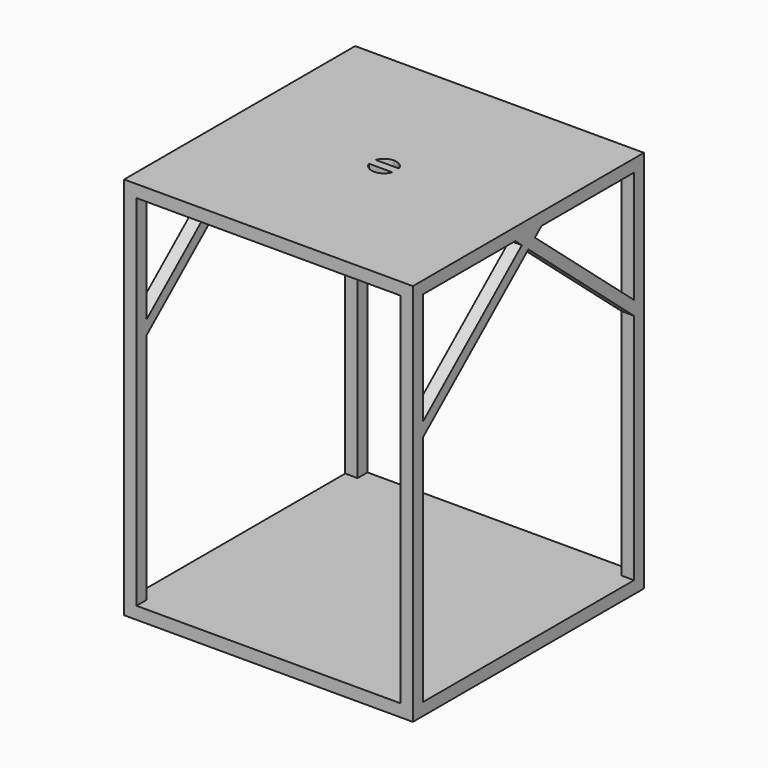
from build123d import *

# Parameters (mm, degrees)
F0_W     = 35
F0_H     = 70
F1_DEPTH = 3
F3_DEPTH = 3
F5_DEPTH = 3


# Not quite as in the source:
# - a feature names something its author has since deleted; it is built from what else it names


with BuildPart() as f1:
    # F0 (on Top) → F1 (new body)
    with BuildSketch(Plane.XY):
        with Locations((-17.5, 35)):
            Rectangle(F0_W, F0_H)
    extrude(amount=F1_DEPTH)

    # F2 (on face) → F3 (join)
    with BuildSketch(Plane(origin=(-35, 0, 0), x_dir=(0, -1, 0), z_dir=(-1, 0, 0))):
        Polygon((-35, 86.622338891), (-3, 59.4277828932), (-3, 62.8054440022), (-33.0127427803, 88.3111694455), align=None)
        Polygon((-67, 62.8054440022), (-67, 59.4277828932), (-35, 86.622338891), (-36.9872572197, 88.3111694455), align=None)
        Polygon((-70, 93), (-70, 90), (-67, 90), (-38.9745144394, 90), (-35, 90), (-35, 93), align=None)
        Polygon((0, 93), (-35, 93), (-35, 90), (-31.0254855606, 90), (-3, 90), (0, 90), align=None)
        Polygon((-35, 90), (-33.0127427803, 88.3111694455), (-31.0254855606, 90), align=None)
        Polygon((-36.9872572197, 88.3111694455), (-35, 86.622338891), (-33.0127427803, 88.3111694455), (-35, 90), align=None)
        Polygon((-35, 90), (-38.9745144394, 90), (-36.9872572197, 88.3111694455), align=None)
        Polygon((-70, 90), (-70, 3), (-67, 3), (-67, 59.4277828932), (-67, 62.8054440022), (-67, 90), align=None)
        Polygon((-3, 59.4277828932), (-3, 3), (0, 3), (0, 90), (-3, 90), (-3, 62.8054440022), align=None)
    extrude(amount=-F3_DEPTH)

    # F4 (on face) → F5 (join)
    with BuildSketch(Plane.XY.offset(93)):
        with BuildLine():
            Line((-32, 70), (-32, 0))
            Line((-32, 0), (0, 0))
            Line((0, 0), (0, 32))
            ThreePointArc((0, 32), (-1.7320508076, 32.5505102572), (-2.8284271247, 34))
            ThreePointArc((-2.8284271247, 34), (-3, 35), (-2.8284271247, 36))
            ThreePointArc((-2.8284271247, 36), (-1.7320508076, 37.4494897428), (0, 38))
            Line((0, 38), (0, 70))
            Line((0, 70), (-32, 70))
        make_face()
        with BuildLine():
            Line((-2.8284271247, 34), (0, 34))
            Line((0, 34), (0, 36))
            Line((0, 36), (-2.8284271247, 36))
            ThreePointArc((-2.8284271247, 36), (-3, 35), (-2.8284271247, 34))
        make_face()
    extrude(amount=-F5_DEPTH)

    # F6: F1 across plane


with BuildPart() as f1_1:
    add(f1.part)
    add(f1.part.mirror(Plane.YZ))


solid = f1_1.part
